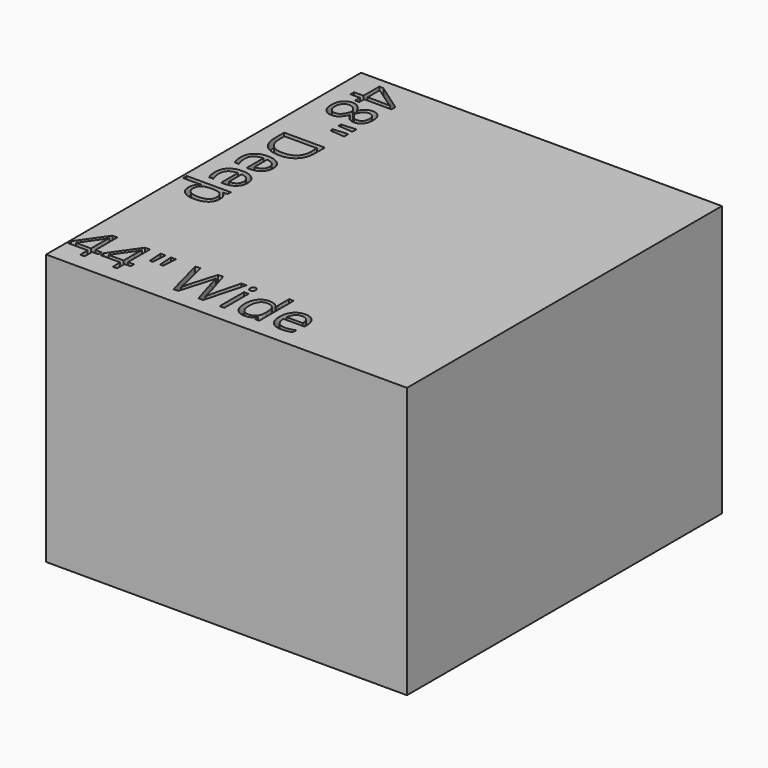
from build123d import *

# Parameters (mm, degrees)
F0_W         = 1117.6
F0_H         = 1219.2
F1_DEPTH     = 838.2
F2_TEXT_SIZE = 176.3888888889
F3_DEPTH     = 25.4


# Not quite as in the source:
# - Text() gives the source's letters only with a copy of the font that has no kerning and outlines rounded to 1/6400 em; it was checked with that copy


with BuildPart() as f1:
    # F0 (on Top) → F1 (new body)
    with BuildSketch(Plane.XY):
        Rectangle(F0_W, F0_H)
    extrude(amount=F1_DEPTH)

    # F2 (on face) → F3 (cut)
    with BuildSketch(Plane.XY.offset(838.2)):
        with Locations((-558.8, -558.8)):
            Text('44" Wide', F2_TEXT_SIZE, font='Open Sans', text_align=(TextAlign.LEFT, TextAlign.BOTTOM))
        with Locations(Location((-508, 584.2), (0, 0, -90))):
            Text('48" Deep', F2_TEXT_SIZE, font='Open Sans', text_align=(TextAlign.LEFT, TextAlign.BOTTOM))
    extrude(amount=-F3_DEPTH, mode=Mode.SUBTRACT)


solid = f1.part
